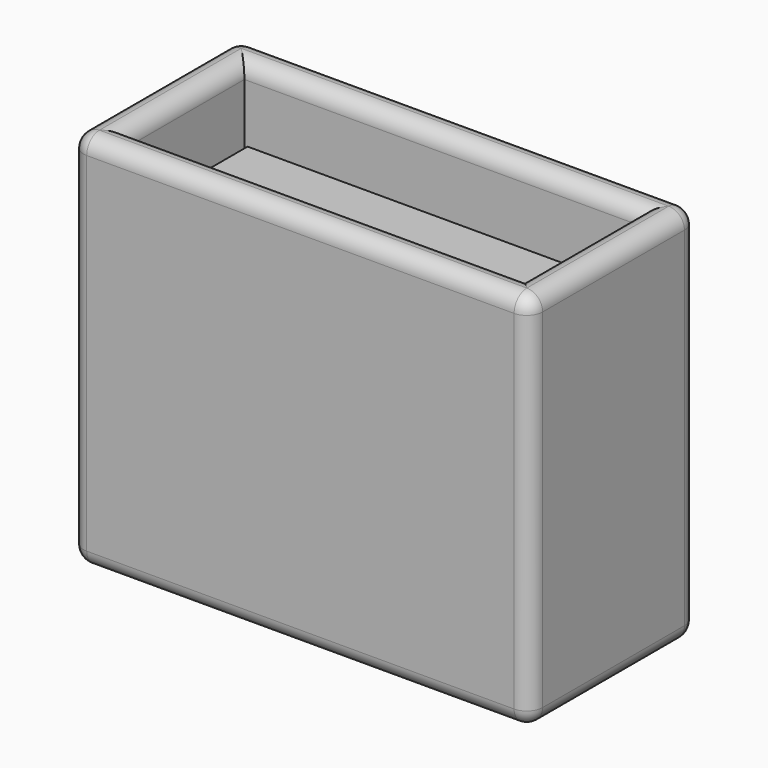
from build123d import *

# Parameters (mm, degrees)
F0_W     = 14.5
F0_H     = 6.6
F0_W_2   = 12.5
F0_H_2   = 4.6
F1_DEPTH = 12
F0_W_3   = 11.5
F0_H_3   = 1.7
F2_DEPTH = 2
F3_DEPTH = 10
F4_R     = 0.49999
F6_DEPTH = 0.4


# Not quite as in the source:
# - a fillet or chamfer is up to 0.001 mm smaller than in the source, because OpenCascade refuses the exact size


with BuildPart() as f1:
    # F0 (on Top) → F1 (new body)
    with BuildSketch(Plane.XY):
        with Locations((0.6113282288, 0)):
            Rectangle(F0_W, F0_H)
        with Locations((0.6113282288, 0)):
            Rectangle(F0_W_2, F0_H_2, mode=Mode.SUBTRACT)
    extrude(amount=F1_DEPTH)

    # F0 (on Top) → F2 (join)
    with BuildSketch(Plane.XY):
        with Locations((0.6113282288, 0)):
            Rectangle(F0_W_2, F0_H_2)
        with Locations((0.6113282288, 0.95)):
            Rectangle(F0_W_3, F0_H_3, mode=Mode.SUBTRACT)
        with Locations((0.6113282288, 0.95)):
            Rectangle(F0_W_3, F0_H_3)
    extrude(amount=F2_DEPTH)

    # F0 (on Top) → F3 (join)
    with BuildSketch(Plane.XY):
        with Locations((0.6113282288, 0.95)):
            Rectangle(F0_W_3, F0_H_3)
    extrude(amount=F3_DEPTH)

    # F4 (radius 0.5 in the source; OpenCascade refuses exactly that, so slightly less here)
    f4_edges = [f1.edges().sort_by_distance(p)[0] for p in [
        (-6.638672, 0, 12),
        (0.611328, -3.3, 12),
        (7.861328, 0, 12),
        (0.611328, 3.3, 12),
        (-5.638672, 0, 12),
        (0.611328, 2.3, 12),
        (6.861328, 0, 12),
        (0.611328, -2.3, 12),
        (7.861328, 3.3, 6),
        (7.861328, -3.3, 6),
        (7.861328, 0, 0),
        (0.611328, 3.3, 0),
        (-6.638672, 3.3, 6),
        (-6.638672, -3.3, 6),
        (0.611328, -3.3, 0),
        (-6.638672, 0, 0),
    ]]
    fillet(f4_edges, radius=F4_R)

    # F5 (on face) → F6 (cut)
    with BuildSketch(Plane(origin=(0, 3.3, 0), x_dir=(-1, 0, 0), z_dir=(0, 1, 0))):
        with BuildLine():
            Line((-4.1945352975, 7.1148852238), (-4.1945352975, 7.3648852238))
            ThreePointArc((-4.1945352975, 7.3648852238), (-6.193634283, 5.4249122664), (-4.3145352975, 3.3684884696))
            Line((-4.3145352975, 3.3684884696), (-4.3145352975, 3.6190043573))
            ThreePointArc((-4.3145352975, 3.6190043573), (-5.9435052109, 5.4249205618), (-4.1945352975, 7.1148852238))
        make_face()
        with BuildLine():
            Line((-4.3145352975, 3.6190043573), (-4.3145352975, 3.3684884696))
            ThreePointArc((-4.3145352975, 3.3684884696), (-4.1895255031, 3.3648914983), (-4.0645352975, 3.3691146959))
            Line((-4.0645352975, 3.3691146959), (-4.0645352975, 3.6197204751))
            ThreePointArc((-4.0645352975, 3.6197204751), (-4.1895224932, 3.6148924033), (-4.3145352975, 3.6190043573))
        make_face()
        with BuildLine():
            ThreePointArc((-4.0645352975, 3.3691146959), (-4.1895255031, 3.3648914983), (-4.3145352975, 3.3684884696))
            Line((-4.3145352975, 3.3684884696), (-4.3145352975, 1.8648852238))
            Line((-4.3145352975, 1.8648852238), (-4.0645352975, 1.8648852238))
            Line((-4.0645352975, 1.8648852238), (-4.0645352975, 3.3691146959))
        make_face()
        with BuildLine():
            Line((-4.0645352975, 3.6197204751), (-4.0645352975, 3.3691146959))
            ThreePointArc((-4.0645352975, 3.3691146959), (-2.7350833455, 3.9974057907), (-2.1945352975, 5.3648852238))
            Line((-2.1945352975, 5.3648852238), (-2.4445352975, 5.3648852238))
            ThreePointArc((-2.4445352975, 5.3648852238), (-2.4490283635, 5.2395634644), (-2.4624844899, 5.1148852238))
            ThreePointArc((-2.4624844899, 5.1148852238), (-3.000513644, 4.0855055729), (-4.0645352975, 3.6197204751))
        make_face()
        with BuildLine():
            Line((-4.3145352975, 5.3648852238), (-4.3145352975, 3.6190043573))
            ThreePointArc((-4.3145352975, 3.6190043573), (-4.1895224932, 3.6148924033), (-4.0645352975, 3.6197204751))
            Line((-4.0645352975, 3.6197204751), (-4.0645352975, 5.1148852238))
            Line((-4.0645352975, 5.1148852238), (-2.4624844899, 5.1148852238))
            ThreePointArc((-2.4624844899, 5.1148852238), (-2.4490283635, 5.2395634644), (-2.4445352975, 5.3648852238))
            Line((-2.4445352975, 5.3648852238), (-4.3145352975, 5.3648852238))
        make_face()
    extrude(amount=-F6_DEPTH, mode=Mode.SUBTRACT)


solid = f1.part
